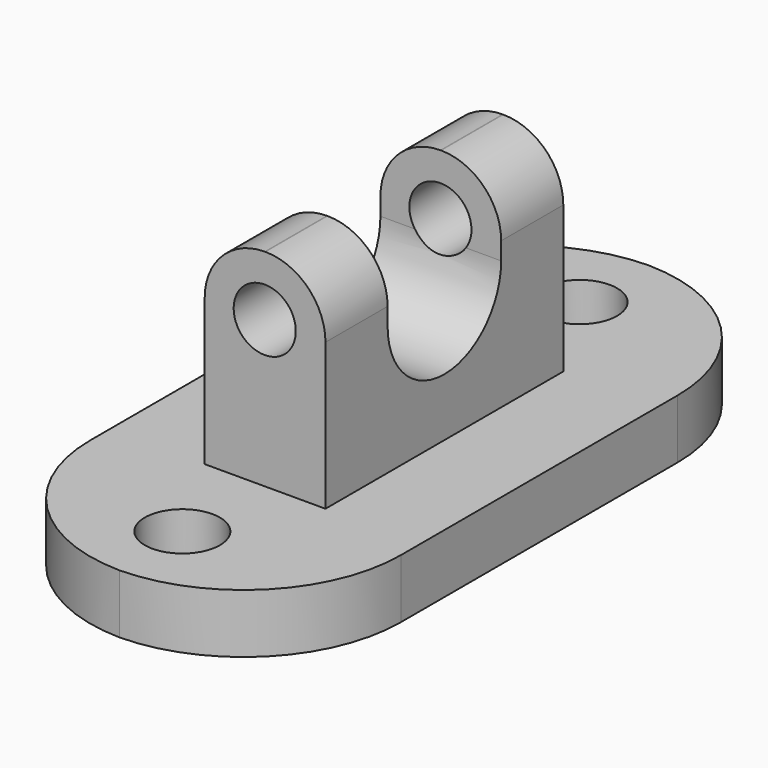
from build123d import *

# Parameters (mm, degrees)
F0_W        = 50.8
F0_H        = 108.0689131842
F1_DEPTH    = 9.652
F2_T1_DEPTH = 138.426151417
F3_R        = 6.1341
F3_R_2      = 6.1313496656
F4_DEPTH    = 9.653
F5_W        = 19.7433687763
F5_H        = 48.6069692673
F6_DEPTH    = 33.782
F7_W        = 23.2069692673
F7_H        = 12.7
F8_DEPTH    = 35.2726834568
F9_R        = 9.8113639175
F10_R       = 5.08
F11_DEPTH   = 78.3378719873


# Not quite as in the source:
# - a fillet or chamfer that OpenCascade refuses, or shapes differently, is made with other operations: its cross-section is extruded or revolved along the edge and cut away or added


with BuildPart() as f1:
    # F0 (on Top) → F1 (new body)
    with BuildSketch(Plane.XY):
        with Locations((0.4926733673, 0)):
            Rectangle(F0_W, F0_H)
    extrude(amount=F1_DEPTH)

    # F2: fillet of radius 25.7548302834 on 4 edges, made by hand

    # F2_s2 → F2_t1 (cut)
    with BuildSketch(Plane.XY.offset(-64.3870757085)):
        with BuildLine():
            ThreePointArc((25.8926733673, 28.2796263087), (18.3492582256, 46.4910414504), (0.1378430839, 54.0344565921))
            Line((0.1378430839, 54.0344565921), (25.8926733673, 54.0344565921))
            Line((25.8926733673, 54.0344565921), (25.8926733673, 28.2796263087))
        make_face()
        with BuildLine():
            ThreePointArc((0.8475036507, 54.0344565921), (-17.363911491, 46.4910414504), (-24.9073266327, 28.2796263087))
            Line((-24.9073266327, 28.2796263087), (-24.9073266327, 54.0344565921))
            Line((-24.9073266327, 54.0344565921), (0.8475036507, 54.0344565921))
        make_face()
        with BuildLine():
            ThreePointArc((0.1378430839, -54.0344565921), (18.3492582256, -46.4910414504), (25.8926733673, -28.2796263087))
            Line((25.8926733673, -28.2796263087), (25.8926733673, -54.0344565921))
            Line((25.8926733673, -54.0344565921), (0.1378430839, -54.0344565921))
        make_face()
        with BuildLine():
            ThreePointArc((0.8475036507, -54.0344565921), (-17.363911491, -46.4910414504), (-24.9073266327, -28.2796263087))
            Line((-24.9073266327, -28.2796263087), (-24.9073266327, -54.0344565921))
            Line((-24.9073266327, -54.0344565921), (0.8475036507, -54.0344565921))
        make_face()
    extrude(amount=F2_T1_DEPTH, mode=Mode.SUBTRACT)

    # F3 (on face) → F4 (cut, through all)
    with BuildSketch(Plane.XY.offset(9.652)):
        with Locations((0, -40.5962094665)):
            Circle(F3_R)
        with Locations((0, 40.5962094665)):
            Circle(F3_R_2)
    extrude(amount=-F4_DEPTH, mode=Mode.SUBTRACT)

    # F5 (on face) → F6 (join)
    with BuildSketch(Plane.XY.offset(9.652)):
        with Locations((0.4926724359, 0.0013751672)):
            Rectangle(F5_W, F5_H)
    extrude(amount=F6_DEPTH)

    # F7 (on face) → F8 (cut, through all)
    with BuildSketch(Plane.YZ.offset(10.3643568241)):
        with Locations((0.0013751672, 37.084)):
            Rectangle(F7_W, F7_H)
        with BuildLine():
            Line((11.6048598008, 30.734), (-11.6021094665, 30.734))
            ThreePointArc((-11.6021094665, 30.734), (0.0013751672, 19.1305153664), (11.6048598008, 30.734))
        make_face()
    extrude(amount=-F8_DEPTH, mode=Mode.SUBTRACT)

    # F9
    f9_edges = [f1.edges().sort_by_distance(p)[0] for p in [
        (-9.379012, 17.95486, 43.434),
        (10.364357, 17.95486, 43.434),
        (-9.379012, -17.952109, 43.434),
        (10.364357, -17.952109, 43.434),
    ]]
    fillet(f9_edges, radius=F9_R)

    # F10 (on face) → F11 (cut, through all)
    with BuildSketch(Plane(origin=(0, 24.3048598008, 0), x_dir=(-1, 0, 0), z_dir=(0, 1, 0))):
        with Locations((-0.4323519653, 33.6226360825)):
            Circle(F10_R)
    extrude(amount=-F11_DEPTH, mode=Mode.SUBTRACT)


solid = f1.part
